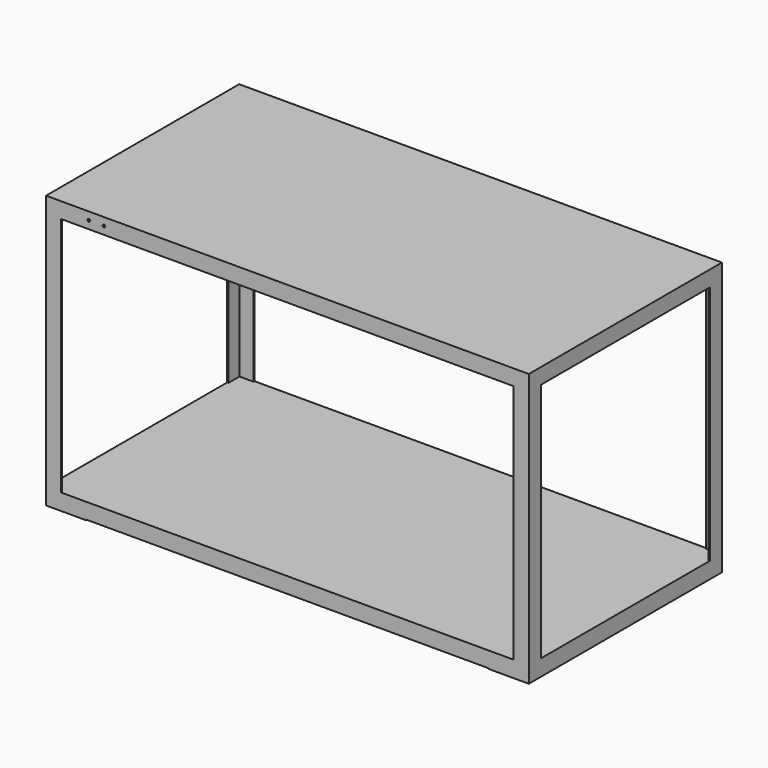
from build123d import *

# Parameters (mm, degrees)
F0_W              = 1219.2
F0_H              = 609.6
F1_DEPTH          = 1.51892
F2_W              = 1219.2
F2_H              = 609.6
F2_W_2            = 1216.16216
F2_H_2            = 606.56216
F3_DEPTH          = 38.1
F5_DEPTH          = 685.8
F7_W              = 1219.2
F7_H              = 609.6
F8_DEPTH          = 1.51892
F9_W              = 1219.2
F9_H              = 609.6
F9_W_2            = 1213.12432
F9_H_2            = 603.52432
F10_DEPTH         = 38.1
F11_W             = 101.6
F11_H             = 609.6
F12_DEPTH         = 1.51892
F13_R             = 1.5875
F14_DEPTH         = 1.651
F14_COPIES2_COUNT = 2
F14_COPIES2_PITCH = 1240.259203
F16_D             = 6.35


# Not quite as in the source:
# - a pattern or mirror of a feature is missing from the dataset's text; its kind, count and spacing are read off the source's solid


with BuildPart() as f1:
    # F0 (on Top) → F1 (new body)
    with BuildSketch(Plane.XY):
        Rectangle(F0_W, F0_H)
    extrude(amount=-F1_DEPTH)

    # F2 (on face) → F3 (join)
    with BuildSketch(Plane(origin=(0, 0, -1.51892), x_dir=(1, 0, 0), z_dir=(0, 0, -1))):
        Rectangle(F2_W, F2_H)
        Rectangle(F2_W_2, F2_H_2, mode=Mode.SUBTRACT)
    extrude(amount=F3_DEPTH)

    # F4 (on face) → F5 (join)
    with BuildSketch(Plane(origin=(0, 0, -1.51892), x_dir=(1, 0, 0), z_dir=(0, 0, -1))):
        Polygon((-571.5, 301.76216), (-571.5, 304.8), (-609.6, 304.8), (-609.6, 266.7), (-606.56216, 266.7), (-606.56216, 301.76216), align=None)
        Polygon((571.5, 304.8), (571.5, 301.76216), (606.56216, 301.76216), (606.56216, 266.7), (609.6, 266.7), (609.6, 304.8), align=None)
    f5 = extrude(amount=F5_DEPTH)

    # F5_copies: F5 across plane
    add(f5.mirror(Plane.ZX))

    # F7 (on offset) → F8 (join)
    with BuildSketch(Plane.XY.offset(-647.7)):
        Rectangle(F7_W, F7_H)
    extrude(amount=-F8_DEPTH)

    # F9 (on face) → F10 (join)
    with BuildSketch(Plane(origin=(0, 0, -649.21892), x_dir=(1, 0, 0), z_dir=(0, 0, -1))):
        Rectangle(F9_W, F9_H)
        Rectangle(F9_W_2, F9_H_2, mode=Mode.SUBTRACT)
    extrude(amount=F10_DEPTH)

    # F11 (on face) → F12 (join)
    with BuildSketch(Plane(origin=(0, 0, -687.31892), x_dir=(1, 0, 0), z_dir=(0, 0, -1))):
        with Locations((-558.8, 0)):
            Rectangle(F11_W, F11_H)
    f12 = extrude(amount=F12_DEPTH)

    # F12_copies: F12 across plane
    add(f12.mirror(Plane(origin=(0, 0, 0), x_dir=(0, 0, 1), z_dir=(1, 0, 0))))

    # F13 (on face) → F14 (cut)
    with BuildSketch(Plane(origin=(0, 0, -688.83784), x_dir=(1, 0, 0), z_dir=(0, 0, -1))):
        with Locations((-596.9, 292.1)):
            Circle(F13_R)
        with Locations((-596.9, 225.425)):
            Circle(F13_R)
        with Locations((-530.225, 292.1)):
            Circle(F13_R)
        with Locations((-530.225, 225.425)):
            Circle(F13_R)
    f14 = extrude(amount=-F14_DEPTH, mode=Mode.SUBTRACT)

    # F14_copies: F14 across plane
    add(f14.mirror(Plane(origin=(0, 0, 0), x_dir=(0, 0, 1), z_dir=(1, 0, 0))), mode=Mode.SUBTRACT)

    # F14_copies1: F14 across plane
    add(f14.mirror(Plane.ZX), mode=Mode.SUBTRACT)

    # F14_copies2: F14 ×2
    with Locations(*[Vector(0.9087818071, 0.4172716466, 0) * (i * F14_COPIES2_PITCH) for i in range(1, F14_COPIES2_COUNT)]):
        add(f14, mode=Mode.SUBTRACT)

    # F16 (through all)
    with Locations(Plane.XZ.offset(304.8)):
        with Locations((-501.65, -19.812), (-463.55, -19.812)):
            Hole(F16_D / 2)


solid = f1.part
